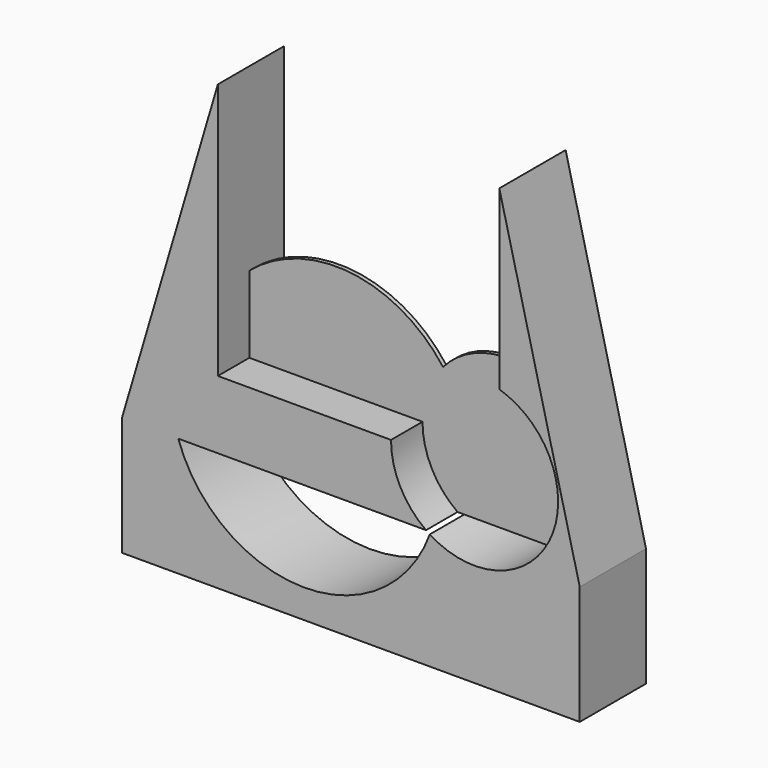
from build123d import *

# Parameters (mm, degrees)
F1_DEPTH = 2.54
F2_DEPTH = 0.127


# Not quite as in the source:
# - a feature names something its author has since deleted; it is built from what else it names


with BuildPart() as f1:
    # F0 (on Front) → F1 (new body, symmetric)
    with BuildSketch(Plane.XZ):
        with BuildLine():
            Line((14.1115041016, 7.2841788642), (17.5840938227, 7.2841788642))
            Line((17.5840938227, 7.2841788642), (12.6545671137, 27.1918801591))
            Line((12.6545671137, 27.1918801591), (12.6545671137, 16.3482450677))
            ThreePointArc((12.6545671137, 16.3482450677), (15.261577361, 14.4943512953), (16.2604214978, 11.4553160965))
            ThreePointArc((16.2604214978, 11.4553160965), (15.6916123075, 9.109243219), (14.1115041016, 7.2841788642))
        make_face()
        with BuildLine():
            Line((-4.5987749709, 27.1918801591), (-10.4762865467, 7.2841788642))
            Line((-10.4762865467, 7.2841788642), (-7.0264551949, 7.2841788642))
            ThreePointArc((-7.0264551949, 7.2841788642), (-7.1794052372, 12.0962388338), (-4.5987749709, 16.1606775766))
            Line((-4.5987749709, 16.1606775766), (-4.5987749709, 27.1918801591))
        make_face()
        with BuildLine():
            ThreePointArc((-4.5987749709, 16.1606775766), (-7.1794052372, 12.0962388338), (-7.0264551949, 7.2841788642))
            Line((-7.0264551949, 7.2841788642), (8.1640722191, 7.2841788642))
            ThreePointArc((8.1640722191, 7.2841788642), (6.5839640132, 9.109243219), (6.0151548229, 11.4553160965))
            Line((6.0151548229, 11.4553160965), (0.7099450795, 11.4553160965))
            Line((0.7099450795, 11.4553160965), (-4.5987749709, 11.4553160965))
            Line((-4.5987749709, 11.4553160965), (-4.5987749709, 16.1606775766))
        make_face()
        with BuildLine():
            Line((-10.4762865467, 7.2841788642), (-10.4762865467, 0))
            Line((-10.4762865467, 0), (17.5840938227, 0))
            Line((17.5840938227, 0), (17.5840938227, 7.2841788642))
            Line((17.5840938227, 7.2841788642), (14.1115041016, 7.2841788642))
            ThreePointArc((14.1115041016, 7.2841788642), (11.2751644394, 6.3345251354), (8.3919880677, 7.1307404918))
            ThreePointArc((8.3919880677, 7.1307404918), (0.6285539733, 1.7598537536), (-7.0264551949, 7.2841788642))
            Line((-7.0264551949, 7.2841788642), (-10.4762865467, 7.2841788642))
        make_face()
        with BuildLine():
            Line((-10.4762865467, 7.2841788642), (-10.4762865467, 0))
            Line((-10.4762865467, 0), (17.5840938227, 0))
            Line((17.5840938227, 0), (17.5840938227, 7.2841788642))
            Line((17.5840938227, 7.2841788642), (14.1115041016, 7.2841788642))
            ThreePointArc((14.1115041016, 7.2841788642), (11.2751644394, 6.3345251354), (8.3919880677, 7.1307404918))
            ThreePointArc((8.3919880677, 7.1307404918), (0.6285539733, 1.7598537536), (-7.0264551949, 7.2841788642))
            Line((-7.0264551949, 7.2841788642), (-10.4762865467, 7.2841788642))
        make_face()
    extrude(amount=F1_DEPTH, both=True)

    # F0 (on Front) → F2 (join, symmetric)
    with BuildSketch(Plane.XZ):
        with BuildLine():
            ThreePointArc((7.2737737734, 14.8184641943), (1.628753339, 18.0658576504), (-4.5987749709, 16.1606775766))
            Line((-4.5987749709, 16.1606775766), (-4.5987749709, 11.4553160965))
            Line((-4.5987749709, 11.4553160965), (0.7099450795, 11.4553160965))
            Line((0.7099450795, 11.4553160965), (6.0151548229, 11.4553160965))
            ThreePointArc((6.0151548229, 11.4553160965), (6.3401167864, 13.250788652), (7.2737737734, 14.8184641943))
        make_face()
        with BuildLine():
            ThreePointArc((7.2737737734, 14.8184641943), (6.3401167864, 13.250788652), (6.0151548229, 11.4553160965))
            Line((6.0151548229, 11.4553160965), (8.7471650108, 11.4553160965))
            ThreePointArc((8.7471650108, 11.4553160965), (8.2016302385, 13.220637488), (7.2737737734, 14.8184641943))
        make_face()
        with BuildLine():
            ThreePointArc((6.0151548229, 11.4553160965), (6.5839640132, 9.109243219), (8.1640722191, 7.2841788642))
            Line((8.1640722191, 7.2841788642), (8.4463453539, 7.2841788642))
            ThreePointArc((8.4463453539, 7.2841788642), (8.7776037503, 8.5930277501), (8.8890353081, 9.9385390058))
            ThreePointArc((8.8890353081, 9.9385390058), (8.8534904982, 10.7002377527), (8.7471650108, 11.4553160965))
            Line((8.7471650108, 11.4553160965), (6.0151548229, 11.4553160965))
        make_face()
        with BuildLine():
            Line((8.4463453539, 7.2841788642), (14.1115041016, 7.2841788642))
            ThreePointArc((14.1115041016, 7.2841788642), (15.6916123075, 9.109243219), (16.2604214978, 11.4553160965))
            ThreePointArc((16.2604214978, 11.4553160965), (15.261577361, 14.4943512953), (12.6545671137, 16.3482450677))
            ThreePointArc((12.6545671137, 16.3482450677), (9.7369184571, 16.3826821662), (7.2737737734, 14.8184641943))
            ThreePointArc((7.2737737734, 14.8184641943), (8.2016302385, 13.220637488), (8.7471650108, 11.4553160965))
            ThreePointArc((8.7471650108, 11.4553160965), (8.8534904982, 10.7002377527), (8.8890353081, 9.9385390058))
            ThreePointArc((8.8890353081, 9.9385390058), (8.7776037503, 8.5930277501), (8.4463453539, 7.2841788642))
        make_face()
    extrude(amount=F2_DEPTH, both=True)


solid = f1.part
